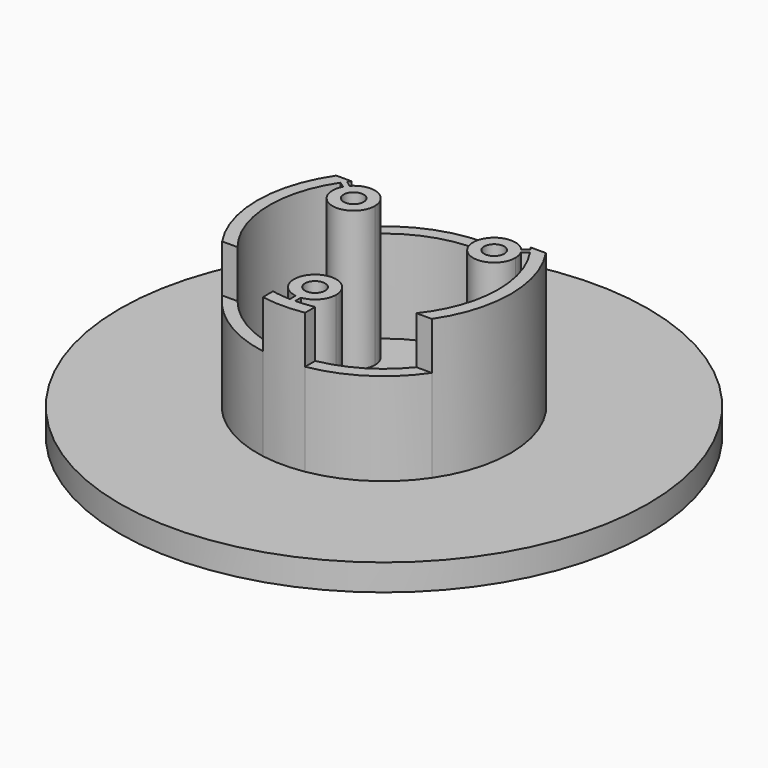
from build123d import *

# Parameters (mm, degrees)
F0_R     = 50
F0_R_2   = 1.9
F1_DEPTH = 5
F2_DEPTH = 17.5
F3_DEPTH = 26.5


# Not quite as in the source:
# - a feature names something its author has since deleted; it is built from what else it names


with BuildPart() as f1:
    # F0 (on Top) → F1 (new body)
    with BuildSketch(Plane.XY):
        Circle(F0_R)
        with BuildLine():
            ThreePointArc((19.843134833, 13.5), (22.9372539332, 7.0627460668), (24, 0))
            ThreePointArc((24, 0), (22.9372539332, -7.0627460668), (19.843134833, -13.5))
            ThreePointArc((19.843134833, -13.5), (12.9596340813, -20.2001951594), (4, -23.6643191324))
            ThreePointArc((4, -23.6643191324), (0, -24), (-4, -23.6643191324))
            ThreePointArc((-4, -23.6643191324), (-12.9596340813, -20.2001951594), (-19.843134833, -13.5))
            ThreePointArc((-19.843134833, -13.5), (-24, 0), (-19.843134833, 13.5))
            ThreePointArc((-19.843134833, 13.5), (0, 24), (19.843134833, 13.5))
        make_face(mode=Mode.SUBTRACT)
        with BuildLine():
            ThreePointArc((4, -23.6643191324), (12.9596340813, -20.2001951594), (19.843134833, -13.5))
            Line((19.843134833, -13.5), (16.9254985156, -13.5))
            ThreePointArc((16.9254985156, -13.5), (11.1620172865, -18.5507916299), (4, -21.2772766114))
            Line((4, -21.2772766114), (4, -23.6643191324))
        make_face()
        with BuildLine():
            ThreePointArc((19.843134833, -13.5), (22.9372539332, -7.0627460668), (24, 0))
            ThreePointArc((24, 0), (22.9372539332, 7.0627460668), (19.843134833, 13.5))
            Line((19.843134833, 13.5), (16.9254985156, 13.5))
            ThreePointArc((16.9254985156, 13.5), (17.1411453437, 13.2251138485), (17.3523282296, 12.9467835778))
            ThreePointArc((17.3523282296, 12.9467835778), (17.6467019836, 12.5425838288), (17.9316623557, 12.1316934169))
            ThreePointArc((17.9316623557, 12.1316934169), (20.6995530145, 6.3443679748), (21.65, 0))
            ThreePointArc((21.65, 0), (20.4347686904, -7.1514144453), (16.9254985156, -13.5))
            Line((16.9254985156, -13.5), (19.843134833, -13.5))
        make_face()
        with BuildLine():
            ThreePointArc((17.3523282296, 12.9467835778), (17.1411453437, 13.2251138485), (16.9254985156, 13.5))
            ThreePointArc((16.9254985156, 13.5), (0, 21.65), (-16.9254985156, 13.5))
            ThreePointArc((-16.9254985156, 13.5), (-17.1411453437, 13.2251138485), (-17.3523282296, 12.9467835778))
            Line((-17.3523282296, 12.9467835778), (-16.2451217298, 12.1598246122))
            ThreePointArc((-16.2451217298, 12.1598246122), (-11.8474999, 13.1800801892), (-9.3, 9.4531184965))
            ThreePointArc((-9.3, 9.4531184965), (-14.2752375549, 5.5738258146), (-16.8244558558, 11.3447344513))
            Line((-16.8244558558, 11.3447344513), (-17.9316623557, 12.1316934169))
            ThreePointArc((-17.9316623557, 12.1316934169), (-21.6333386895, -0.8492097177), (-16.9254985156, -13.5))
            ThreePointArc((-16.9254985156, -13.5), (-11.1620172865, -18.5507916299), (-4, -21.2772766114))
            ThreePointArc((-4, -21.2772766114), (-2.2574682461, -21.5319840497), (-0.5, -21.6442255579))
            Line((-0.5, -21.6442255579), (-0.5, -20.2858402491))
            ThreePointArc((-0.5, -20.2858402491), (-2.6457513111, -13.3172132825), (4, -16.3172132825))
            ThreePointArc((4, -16.3172132825), (3, -18.9629645936), (0.5, -20.2858402491))
            Line((0.5, -20.2858402491), (0.5, -21.6442255579))
            ThreePointArc((0.5, -21.6442255579), (2.2574682461, -21.5319840497), (4, -21.2772766114))
            ThreePointArc((4, -21.2772766114), (11.1620172865, -18.5507916299), (16.9254985156, -13.5))
            ThreePointArc((16.9254985156, -13.5), (20.4347686904, -7.1514144453), (21.65, 0))
            ThreePointArc((21.65, 0), (20.6995530145, 6.3443679748), (17.9316623557, 12.1316934169))
            Line((17.9316623557, 12.1316934169), (16.8244558558, 11.3447344513))
            ThreePointArc((16.8244558558, 11.3447344513), (17.1792926819, 10.4283560513), (17.3, 9.4531184965))
            ThreePointArc((17.3, 9.4531184965), (9.5730383072, 8.0006183965), (16.2451217298, 12.1598246122))
            Line((16.2451217298, 12.1598246122), (17.3523282296, 12.9467835778))
        make_face()
        with BuildLine():
            Line((16.9254985156, 13.5), (19.843134833, 13.5))
            ThreePointArc((19.843134833, 13.5), (0, 24), (-19.843134833, 13.5))
            Line((-19.843134833, 13.5), (-16.9254985156, 13.5))
            ThreePointArc((-16.9254985156, 13.5), (0, 21.65), (16.9254985156, 13.5))
        make_face()
        with BuildLine():
            ThreePointArc((-9.3, 9.4531184965), (-11.8474999, 13.1800801892), (-16.2451217298, 12.1598246122))
            ThreePointArc((-16.2451217298, 12.1598246122), (-16.5603606436, 11.7704550006), (-16.8244558558, 11.3447344513))
            ThreePointArc((-16.8244558558, 11.3447344513), (-14.2752375549, 5.5738258146), (-9.3, 9.4531184965))
        make_face()
        with Locations((-13.3, 9.4531184965)):
            Circle(F0_R_2, mode=Mode.SUBTRACT)
        with BuildLine():
            ThreePointArc((16.8244558558, 11.3447344513), (16.5603606436, 11.7704550006), (16.2451217298, 12.1598246122))
            ThreePointArc((16.2451217298, 12.1598246122), (9.5730383072, 8.0006183965), (17.3, 9.4531184965))
            ThreePointArc((17.3, 9.4531184965), (17.1792926819, 10.4283560513), (16.8244558558, 11.3447344513))
        make_face()
        with Locations((13.3, 9.4531184965)):
            Circle(F0_R_2, mode=Mode.SUBTRACT)
        with BuildLine():
            Line((-16.9254985156, 13.5), (-19.843134833, 13.5))
            ThreePointArc((-19.843134833, 13.5), (-24, 0), (-19.843134833, -13.5))
            Line((-19.843134833, -13.5), (-16.9254985156, -13.5))
            ThreePointArc((-16.9254985156, -13.5), (-21.6333386895, -0.8492097177), (-17.9316623557, 12.1316934169))
            ThreePointArc((-17.9316623557, 12.1316934169), (-17.6467019836, 12.5425838288), (-17.3523282296, 12.9467835778))
            ThreePointArc((-17.3523282296, 12.9467835778), (-17.1411453437, 13.2251138485), (-16.9254985156, 13.5))
        make_face()
        with BuildLine():
            Line((-16.9254985156, -13.5), (-19.843134833, -13.5))
            ThreePointArc((-19.843134833, -13.5), (-12.9596340813, -20.2001951594), (-4, -23.6643191324))
            Line((-4, -23.6643191324), (-4, -21.2772766114))
            ThreePointArc((-4, -21.2772766114), (-11.1620172865, -18.5507916299), (-16.9254985156, -13.5))
        make_face()
        with BuildLine():
            ThreePointArc((-4, -23.6643191324), (0, -24), (4, -23.6643191324))
            Line((4, -23.6643191324), (4, -21.2772766114))
            ThreePointArc((4, -21.2772766114), (2.2574682461, -21.5319840497), (0.5, -21.6442255579))
            ThreePointArc((0.5, -21.6442255579), (0, -21.65), (-0.5, -21.6442255579))
            ThreePointArc((-0.5, -21.6442255579), (-2.2574682461, -21.5319840497), (-4, -21.2772766114))
            Line((-4, -21.2772766114), (-4, -23.6643191324))
        make_face()
        with BuildLine():
            ThreePointArc((-0.5, -20.2858402491), (0, -20.3172132825), (0.5, -20.2858402491))
            ThreePointArc((0.5, -20.2858402491), (3, -18.9629645936), (4, -16.3172132825))
            ThreePointArc((4, -16.3172132825), (-2.6457513111, -13.3172132825), (-0.5, -20.2858402491))
        make_face()
        with Locations((0, -16.3172132825)):
            Circle(F0_R_2, mode=Mode.SUBTRACT)
        with BuildLine():
            ThreePointArc((-0.5, -21.6442255579), (0, -21.65), (0.5, -21.6442255579))
            Line((0.5, -21.6442255579), (0.5, -20.2858402491))
            ThreePointArc((0.5, -20.2858402491), (0, -20.3172132825), (-0.5, -20.2858402491))
            Line((-0.5, -20.2858402491), (-0.5, -21.6442255579))
        make_face()
        with BuildLine():
            ThreePointArc((17.9316623557, 12.1316934169), (17.6467019836, 12.5425838288), (17.3523282296, 12.9467835778))
            Line((17.3523282296, 12.9467835778), (16.2451217298, 12.1598246122))
            ThreePointArc((16.2451217298, 12.1598246122), (16.5603606436, 11.7704550006), (16.8244558558, 11.3447344513))
            Line((16.8244558558, 11.3447344513), (17.9316623557, 12.1316934169))
        make_face()
        with BuildLine():
            Line((-16.2451217298, 12.1598246122), (-17.3523282296, 12.9467835778))
            ThreePointArc((-17.3523282296, 12.9467835778), (-17.6467019836, 12.5425838288), (-17.9316623557, 12.1316934169))
            Line((-17.9316623557, 12.1316934169), (-16.8244558558, 11.3447344513))
            ThreePointArc((-16.8244558558, 11.3447344513), (-16.5603606436, 11.7704550006), (-16.2451217298, 12.1598246122))
        make_face()
    extrude(amount=-F1_DEPTH)

    # F0 (on Top) → F2 (join)
    with BuildSketch(Plane.XY):
        with BuildLine():
            ThreePointArc((4, -23.6643191324), (12.9596340813, -20.2001951594), (19.843134833, -13.5))
            Line((19.843134833, -13.5), (16.9254985156, -13.5))
            ThreePointArc((16.9254985156, -13.5), (11.1620172865, -18.5507916299), (4, -21.2772766114))
            Line((4, -21.2772766114), (4, -23.6643191324))
        make_face()
        with BuildLine():
            Line((-16.9254985156, -13.5), (-19.843134833, -13.5))
            ThreePointArc((-19.843134833, -13.5), (-12.9596340813, -20.2001951594), (-4, -23.6643191324))
            Line((-4, -23.6643191324), (-4, -21.2772766114))
            ThreePointArc((-4, -21.2772766114), (-11.1620172865, -18.5507916299), (-16.9254985156, -13.5))
        make_face()
        with BuildLine():
            Line((16.9254985156, 13.5), (19.843134833, 13.5))
            ThreePointArc((19.843134833, 13.5), (0, 24), (-19.843134833, 13.5))
            Line((-19.843134833, 13.5), (-16.9254985156, 13.5))
            ThreePointArc((-16.9254985156, 13.5), (0, 21.65), (16.9254985156, 13.5))
        make_face()
    extrude(amount=F2_DEPTH)

    # F0 (on Top) → F3 (join)
    with BuildSketch(Plane.XY):
        with BuildLine():
            Line((-16.9254985156, 13.5), (-19.843134833, 13.5))
            ThreePointArc((-19.843134833, 13.5), (-24, 0), (-19.843134833, -13.5))
            Line((-19.843134833, -13.5), (-16.9254985156, -13.5))
            ThreePointArc((-16.9254985156, -13.5), (-21.6333386895, -0.8492097177), (-17.9316623557, 12.1316934169))
            ThreePointArc((-17.9316623557, 12.1316934169), (-17.6467019836, 12.5425838288), (-17.3523282296, 12.9467835778))
            ThreePointArc((-17.3523282296, 12.9467835778), (-17.1411453437, 13.2251138485), (-16.9254985156, 13.5))
        make_face()
        with BuildLine():
            ThreePointArc((19.843134833, -13.5), (22.9372539332, -7.0627460668), (24, 0))
            ThreePointArc((24, 0), (22.9372539332, 7.0627460668), (19.843134833, 13.5))
            Line((19.843134833, 13.5), (16.9254985156, 13.5))
            ThreePointArc((16.9254985156, 13.5), (17.1411453437, 13.2251138485), (17.3523282296, 12.9467835778))
            ThreePointArc((17.3523282296, 12.9467835778), (17.6467019836, 12.5425838288), (17.9316623557, 12.1316934169))
            ThreePointArc((17.9316623557, 12.1316934169), (20.6995530145, 6.3443679748), (21.65, 0))
            ThreePointArc((21.65, 0), (20.4347686904, -7.1514144453), (16.9254985156, -13.5))
            Line((16.9254985156, -13.5), (19.843134833, -13.5))
        make_face()
        with BuildLine():
            ThreePointArc((16.8244558558, 11.3447344513), (16.5603606436, 11.7704550006), (16.2451217298, 12.1598246122))
            ThreePointArc((16.2451217298, 12.1598246122), (9.5730383072, 8.0006183965), (17.3, 9.4531184965))
            ThreePointArc((17.3, 9.4531184965), (17.1792926819, 10.4283560513), (16.8244558558, 11.3447344513))
        make_face()
        with Locations((13.3, 9.4531184965)):
            Circle(F0_R_2, mode=Mode.SUBTRACT)
        with BuildLine():
            ThreePointArc((-0.5, -20.2858402491), (0, -20.3172132825), (0.5, -20.2858402491))
            ThreePointArc((0.5, -20.2858402491), (3, -18.9629645936), (4, -16.3172132825))
            ThreePointArc((4, -16.3172132825), (-2.6457513111, -13.3172132825), (-0.5, -20.2858402491))
        make_face()
        with Locations((0, -16.3172132825)):
            Circle(F0_R_2, mode=Mode.SUBTRACT)
        with BuildLine():
            ThreePointArc((-0.5, -21.6442255579), (0, -21.65), (0.5, -21.6442255579))
            Line((0.5, -21.6442255579), (0.5, -20.2858402491))
            ThreePointArc((0.5, -20.2858402491), (0, -20.3172132825), (-0.5, -20.2858402491))
            Line((-0.5, -20.2858402491), (-0.5, -21.6442255579))
        make_face()
        with BuildLine():
            ThreePointArc((-4, -23.6643191324), (0, -24), (4, -23.6643191324))
            Line((4, -23.6643191324), (4, -21.2772766114))
            ThreePointArc((4, -21.2772766114), (2.2574682461, -21.5319840497), (0.5, -21.6442255579))
            ThreePointArc((0.5, -21.6442255579), (0, -21.65), (-0.5, -21.6442255579))
            ThreePointArc((-0.5, -21.6442255579), (-2.2574682461, -21.5319840497), (-4, -21.2772766114))
            Line((-4, -21.2772766114), (-4, -23.6643191324))
        make_face()
        with BuildLine():
            ThreePointArc((-9.3, 9.4531184965), (-11.8474999, 13.1800801892), (-16.2451217298, 12.1598246122))
            ThreePointArc((-16.2451217298, 12.1598246122), (-16.5603606436, 11.7704550006), (-16.8244558558, 11.3447344513))
            ThreePointArc((-16.8244558558, 11.3447344513), (-14.2752375549, 5.5738258146), (-9.3, 9.4531184965))
        make_face()
        with Locations((-13.3, 9.4531184965)):
            Circle(F0_R_2, mode=Mode.SUBTRACT)
        with BuildLine():
            Line((-16.2451217298, 12.1598246122), (-17.3523282296, 12.9467835778))
            ThreePointArc((-17.3523282296, 12.9467835778), (-17.6467019836, 12.5425838288), (-17.9316623557, 12.1316934169))
            Line((-17.9316623557, 12.1316934169), (-16.8244558558, 11.3447344513))
            ThreePointArc((-16.8244558558, 11.3447344513), (-16.5603606436, 11.7704550006), (-16.2451217298, 12.1598246122))
        make_face()
        with BuildLine():
            ThreePointArc((17.9316623557, 12.1316934169), (17.6467019836, 12.5425838288), (17.3523282296, 12.9467835778))
            Line((17.3523282296, 12.9467835778), (16.2451217298, 12.1598246122))
            ThreePointArc((16.2451217298, 12.1598246122), (16.5603606436, 11.7704550006), (16.8244558558, 11.3447344513))
            Line((16.8244558558, 11.3447344513), (17.9316623557, 12.1316934169))
        make_face()
    extrude(amount=F3_DEPTH)


solid = f1.part
